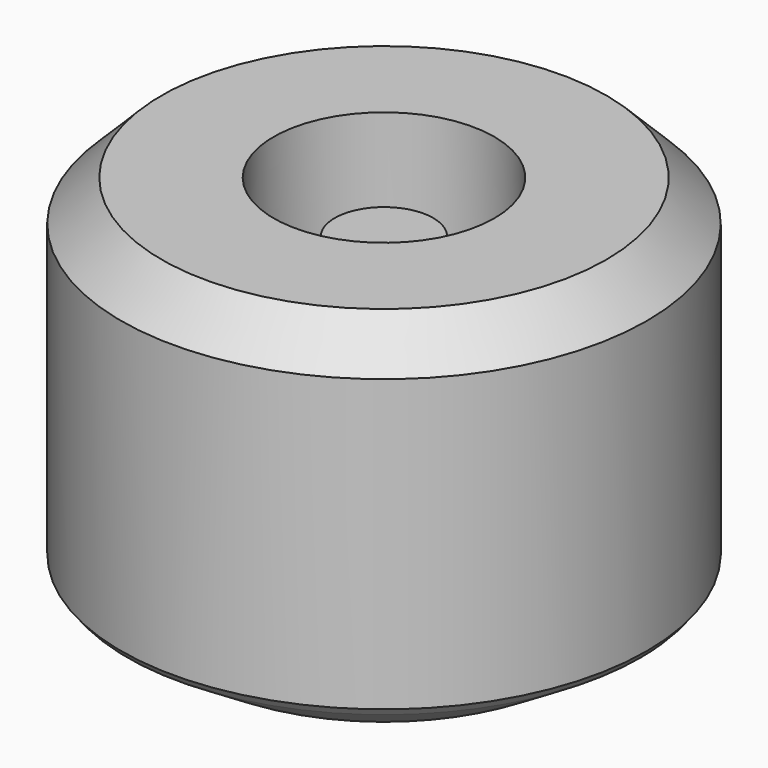
from build123d import *

# Parameters (mm, degrees)
F3_SIZE = 5.08


# Not quite as in the source:
# - a fillet or chamfer that OpenCascade refuses, or shapes differently, is made with other operations: its cross-section is extruded or revolved along the edge and cut away or added


with BuildPart() as f1:
    # F0 (on Front) → F1 (revolve)
    with BuildSketch(Plane.XZ):
        Polygon((32.8848399222, 52.7038350701), (13.7998890132, 52.7038350701), (13.7998890132, 35.9677970409), (6.1659086496, 35.9677970409), (6.1659086496, 46.2443120778), (0, 46.2443120778), (0, 0), (32.8848399222, 7.1935597807), align=None)
    revolve(axis=Axis((0, 0, 23.1221560389), (0, 0, -1)))

    # F2: chamfer of 5.08 on 3 edges, made by hand

    # F2_s1 → F2_t2 (revolve, cut)
    with BuildSketch(Plane.XZ):
        Polygon((28.8904202174, 6.319780343), (32.8848399222, 11.2824323984), (32.8848399222, 7.1935597807), align=None)
    revolve(axis=Axis((0, 0, 7.1935597807), (0, 0, -1)), mode=Mode.SUBTRACT)

    # F2_s3 → F2_t4 (revolve, cut)
    with BuildSketch(Plane.XZ):
        Polygon((27.8048399222, 52.7038350701), (32.8848399222, 47.6238350701), (32.8848399222, 52.7038350701), align=None)
    revolve(axis=Axis((0, 0, 52.7038350701), (0, 0, -1)), mode=Mode.SUBTRACT)

    # F3
    f3_edges = [f1.edges().sort_by_distance(p)[0] for p in [
        (14.44521, 0, 3.15989),
        (-28.89042, 0, 6.31978),
    ]]
    chamfer(f3_edges, length=F3_SIZE)


solid = f1.part
